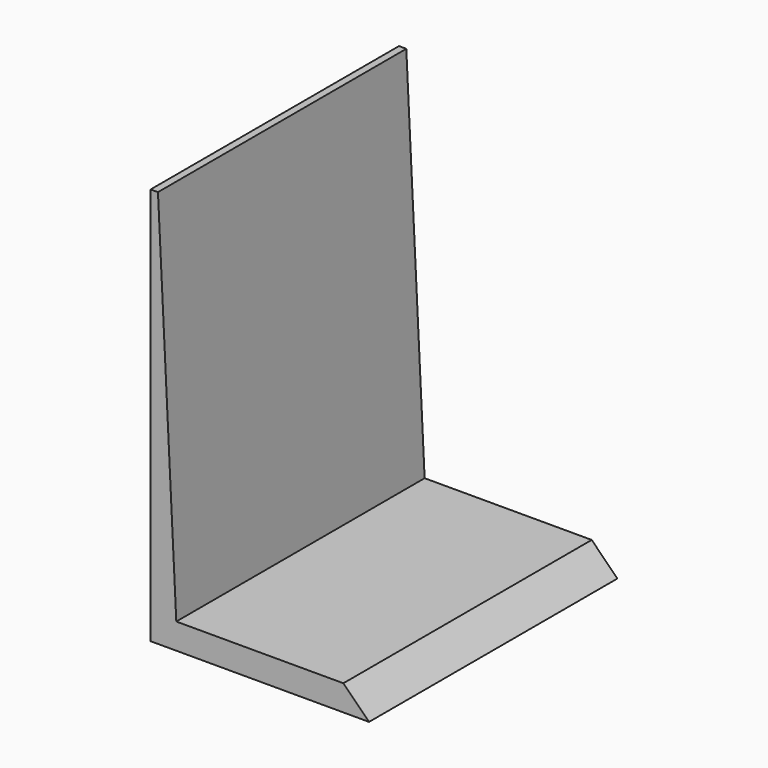
from build123d import *

# Parameters (mm, degrees)
F1_DEPTH    = 86.19552
F3_DEPTH    = 86.19652
F4_T1_DEPTH = 131.920043526


# Not quite as in the source:
# - a fillet or chamfer that OpenCascade refuses, or shapes differently, is made with other operations: its cross-section is extruded or revolved along the edge and cut away or added


with BuildPart() as f1:
    # F0 (on Front) → F1 (new body)
    with BuildSketch(Plane.XZ):
        Polygon((7.1333632804, 110.441185534), (0, 110.441185534), (0, 0), (62.41620332, 0), (62.41620332, 7.1333632804), (7.1333632804, 7.1333632804), align=None)
    extrude(amount=-F1_DEPTH)

    # F2 (on face) → F3 (cut, through all)
    with BuildSketch(Plane.XZ):
        Polygon((7.1333632804, 110.441185534), (7.1333632804, 7.1333632804), (25.2087078989, 24.2729913443), (25.2087078989, 110.441185534), align=None)
        Polygon((2.0419980865, 110.441185534), (7.1333632804, 7.1333632804), (7.1333632804, 110.441185534), align=None)
    extrude(amount=-F3_DEPTH, mode=Mode.SUBTRACT)

    # F4: chamfer of 8.89 on 1 edges, made by hand

    # F4_s2 → F4_t1 (cut)
    with BuildSketch(Plane.XZ.offset(-109.057781763)):
        Polygon((53.52620332, 7.1333632804), (62.41620332, -1.7566367196), (62.41620332, 7.1333632804), align=None)
    extrude(amount=F4_T1_DEPTH, mode=Mode.SUBTRACT)


solid = f1.part
